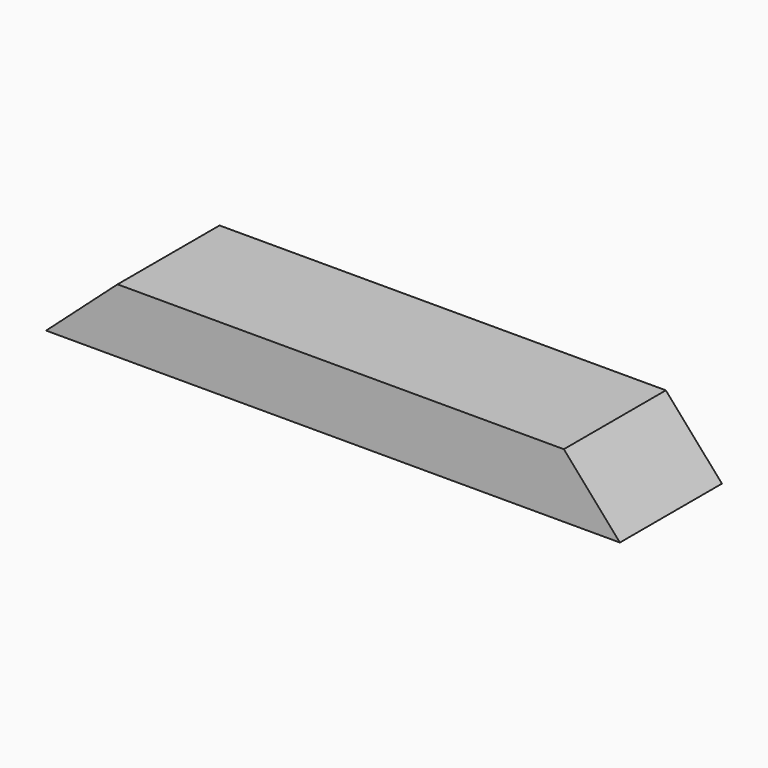
from build123d import *

# Parameters (mm, degrees)
F2_W = 177.8
F2_H = 50.8
F0_W = 228.6
F0_H = 50.8


# Not quite as in the source:
# - the program builds the solid bodies; features that only make, move or delete a surface that nothing else refers to are left out


with BuildPart() as f3:
    # F2 (on offset) → F3 section 0
    with BuildSketch(Plane.XY.offset(25.4)):
        with Locations((18.4815449747, -28.4664724022)):
            Rectangle(F2_W, F2_H)
    # F0 (on Top) → F3 section 1
    with BuildSketch(Plane.XY):
        with Locations((15.5114542365, -28.5803195664)):
            Rectangle(F0_W, F0_H)
    loft()


solid = f3.part
